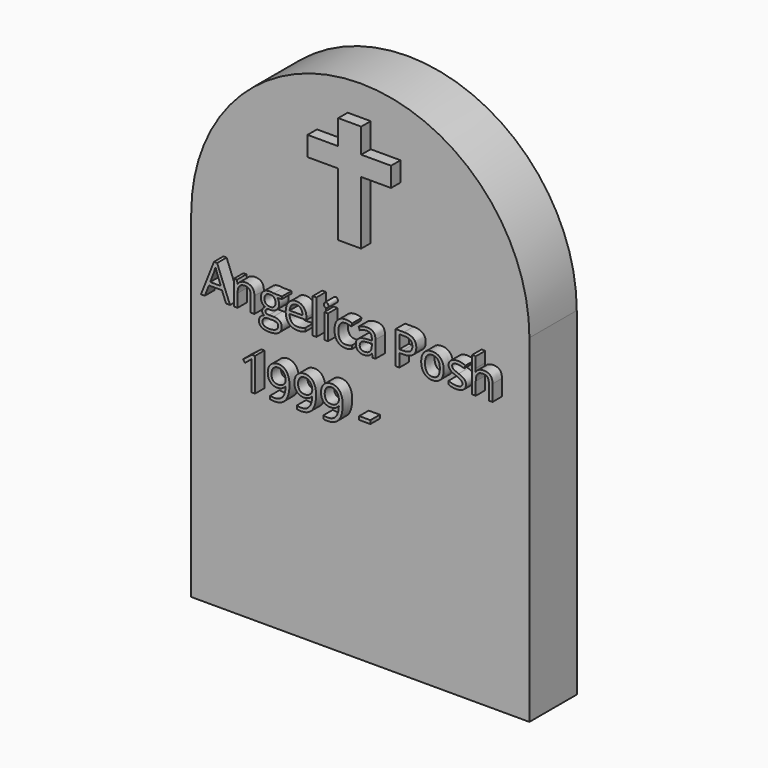
from build123d import *

# Parameters (mm, degrees)
F1_DEPTH       = 17.78
F2_TEXT_SIZE   = 13.7481958114
F2_TEXT_SIZE_2 = 13.9905579595
F3_DEPTH       = 3.556


# Not quite as in the source:
# - Text() gives the source's letters only with a copy of the font that has no kerning and outlines rounded to 1/6400 em; it was checked with that copy


with BuildPart() as f1:
    # F0 (on Front) → F1 (new body)
    with BuildSketch(Plane.XZ):
        with BuildLine():
            Line((-101.6, -101.6), (0, -101.6))
            Line((0, -101.6), (0, 0))
            ThreePointArc((0, 0), (-50.8, 50.8), (-101.6, 0))
            Line((-101.6, 0), (-101.6, -101.6))
        make_face()
    extrude(amount=F1_DEPTH)

    # F2 (on face) → F3 (join)
    with BuildSketch(Plane.XZ.offset(17.78)):
        Polygon((-47.6868003607, 41.792485863), (-54.601944983, 41.792485863), (-54.601944983, 34.3651100993), (-63.8221353292, 34.3651100993), (-63.8221353292, 28.4744352102), (-54.601944983, 28.4744352102), (-54.601944983, 9.5218215138), (-47.6868003607, 9.5218215138), (-47.6868003607, 28.4744352102), (-38.7227274477, 28.4744352102), (-38.7227274477, 34.3651100993), (-47.6868003607, 34.3651100993), align=None)
        with Locations((-95.8197424188, -18.2150120381)):
            Text('Angelica Posh', F2_TEXT_SIZE, font='Open Sans', text_align=(TextAlign.LEFT, TextAlign.BOTTOM))
        with Locations((-84.4933018088, -39.2260961235)):
            Text('1999 -', F2_TEXT_SIZE_2, font='Open Sans', text_align=(TextAlign.LEFT, TextAlign.BOTTOM))
    extrude(amount=F3_DEPTH)


solid = f1.part
